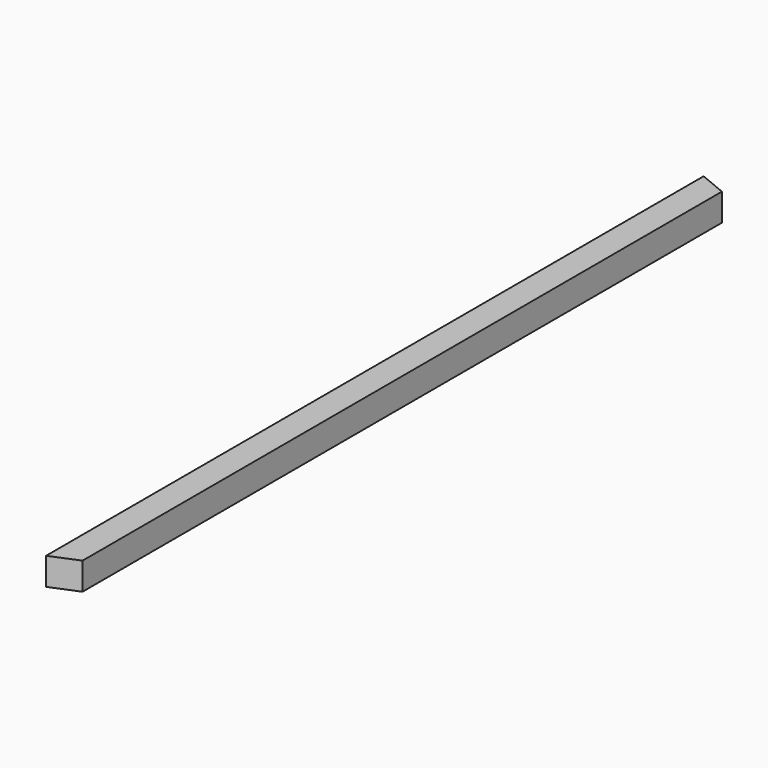
from build123d import *

# Parameters (mm, degrees)
F0_W       = 25.4
F0_H       = 25.4
F1_DEPTH   = 381
F2_SIZE2   = 10.521014
F2_SIZE    = 25.39999
F2_2_SIZE2 = 10.521014
F2_2_SIZE  = 25.39999


# Not quite as in the source:
# - a fillet or chamfer is up to 0.001 mm smaller than in the source, because OpenCascade refuses the exact size


with BuildPart() as f1:
    # F0 (on Front) → F1 (new body, symmetric)
    with BuildSketch(Plane.XZ):
        Rectangle(F0_W, F0_H)
    extrude(amount=F1_DEPTH, both=True)

    # F2 (size 25.4 and 10.5210244843 in the source; OpenCascade refuses exactly that, so slightly less here)
    f2_edges = [f1.edges().sort_by_distance(p)[0] for p in [
        (12.7, -381, 0),
    ]]
    f2_side = f1.faces().sort_by_distance((0, -381, 0))[0]
    chamfer(f2_edges, length=F2_SIZE, length2=F2_SIZE2, reference=f2_side)

    # F2#2 (size 25.4 and 10.5210244843 in the source; OpenCascade refuses exactly that, so slightly less here)
    f2_2_edges = [f1.edges().sort_by_distance(p)[0] for p in [
        (12.7, 381, 0),
    ]]
    f2_2_side = f1.faces().sort_by_distance((0, 381, 0))[0]
    chamfer(f2_2_edges, length=F2_2_SIZE, length2=F2_2_SIZE2, reference=f2_2_side)


solid = f1.part
